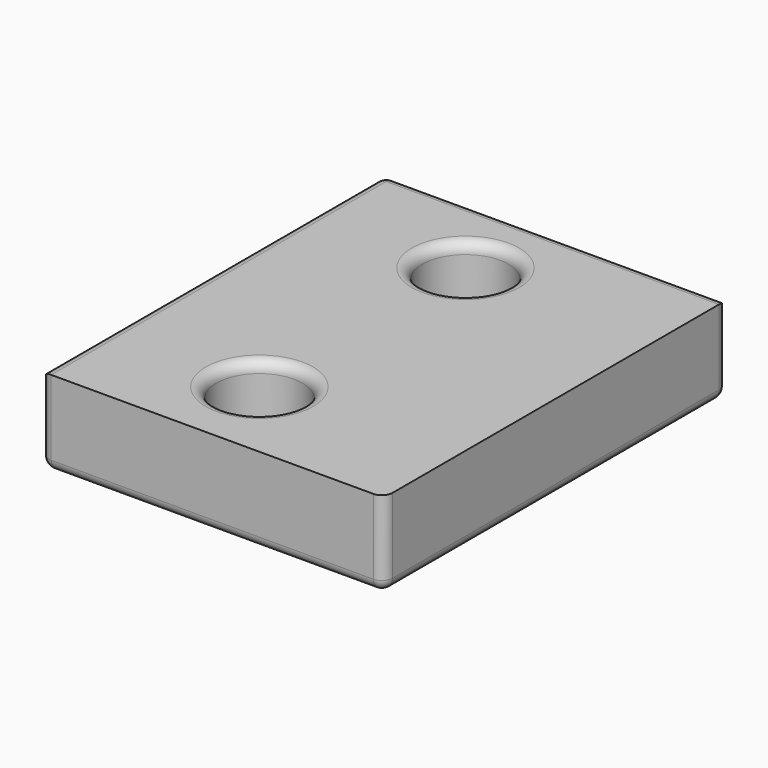
from build123d import *

# Parameters (mm, degrees)
F0_W         = 203.2
F0_H         = 254
F0_R         = 25.4
F1_DEPTH     = 50.8
F2_R         = 6.35
F3_T1_DEPTH  = 53.975
F3_T3_DEPTH  = 60.325
F3_S7_W      = 6.477
F3_S7_H      = 6.477
F3_T8_DEPTH  = 6.477
F3_S13_W     = 6.477
F3_S13_H     = 6.477
F3_T14_DEPTH = 6.477


# Not quite as in the source:
# - a fillet or chamfer that OpenCascade refuses, or shapes differently, is made with other operations: its cross-section is extruded or revolved along the edge and cut away or added


with BuildPart() as f1:
    # F0 (on Top) → F1 (new body)
    with BuildSketch(Plane.XY):
        with Locations((101.6, 127)):
            Rectangle(F0_W, F0_H)
        with Locations((88.8597142273, 50.8)):
            Circle(F0_R, mode=Mode.SUBTRACT)
        with Locations((88.8597142273, 203.2)):
            Circle(F0_R, mode=Mode.SUBTRACT)
    extrude(amount=F1_DEPTH)

    # F2
    f2_edges = [f1.edges().sort_by_distance(p)[0] for p in [
        (0, 127, 0),
        (0, 127, 50.8),
        (101.6, 254, 50.8),
        (63.459714, 203.2, 50.8),
        (63.459714, 50.8, 50.8),
        (101.6, 254, 0),
        (0, 254, 25.4),
        (203.2, 254, 25.4),
        (63.459714, 203.2, 0),
        (63.459714, 50.8, 0),
        (101.6, 0, 0),
        (203.2, 127, 0),
    ]]
    fillet(f2_edges, radius=F2_R)

    # F3: fillet of radius 6.35 on 6 edges, made by hand

    # F3_s2 → F3_t1 (cut)
    with BuildSketch(Plane.XY.offset(6.35)):
        with BuildLine():
            ThreePointArc((0, 6.35), (1.8598719395, 1.8598719395), (6.35, 0))
            Line((6.35, 0), (0, 0))
            Line((0, 0), (0, 6.35))
        make_face()
    extrude(amount=F3_T1_DEPTH, mode=Mode.SUBTRACT)

    # F3_s4 → F3_t3 (cut)
    with BuildSketch(Plane.XY.offset(6.35)):
        with BuildLine():
            ThreePointArc((196.85, 0), (201.3401280605, 1.8598719395), (203.2, 6.35))
            Line((203.2, 6.35), (203.2, 0))
            Line((203.2, 0), (196.85, 0))
        make_face()
    extrude(amount=F3_T3_DEPTH, mode=Mode.SUBTRACT)


with BuildPart() as f3_tool6:
    # F3_s7 → F3_t8 (new body)
    with BuildSketch(Plane.YZ.offset(6.35)):
        with Locations((3.1115, 3.1115)):
            Rectangle(F3_S7_W, F3_S7_H)
    extrude(amount=-F3_T8_DEPTH)

    # F3_s9 → F3_t10 (revolve, cut)
    with BuildSketch(Plane(origin=(6.35, 6.35, 6.35), x_dir=(0, 0.7071067812, 0.7071067812), z_dir=(0, -0.7071067812, 0.7071067812))):
        with BuildLine():
            ThreePointArc((0, -6.35), (6.35, 0), (0, 6.35))
            Line((0, 6.35), (0, -6.35))
        make_face()
    revolve(axis=Axis((6.35, 6.35, 6.35), (-1, 0, 0)), mode=Mode.SUBTRACT)


with BuildPart() as f1_1:
    add(f1.part)

    # F3_t5: cut F3_tool6
    add(f3_tool6.part, mode=Mode.SUBTRACT)


with BuildPart() as f3_tool12:
    # F3_s13 → F3_t14 (new body)
    with BuildSketch(Plane.XZ.offset(-6.35)):
        with Locations((200.0885, 3.1115)):
            Rectangle(F3_S13_W, F3_S13_H)
    extrude(amount=F3_T14_DEPTH)

    # F3_s15 → F3_t16 (revolve, cut)
    with BuildSketch(Plane(origin=(196.85, 6.35, 6.35), x_dir=(-0.7071067812, 0, 0.7071067812), z_dir=(0.7071067812, 0, 0.7071067812))):
        with BuildLine():
            ThreePointArc((0, -6.35), (6.35, 0), (0, 6.35))
            Line((0, 6.35), (0, -6.35))
        make_face()
    revolve(axis=Axis((196.85, 6.35, 6.35), (0, -1, 0)), mode=Mode.SUBTRACT)


with BuildPart() as f1_2:
    add(f1_1.part)

    # F3_t11: cut F3_tool12
    add(f3_tool12.part, mode=Mode.SUBTRACT)


solid = f1_2.part
